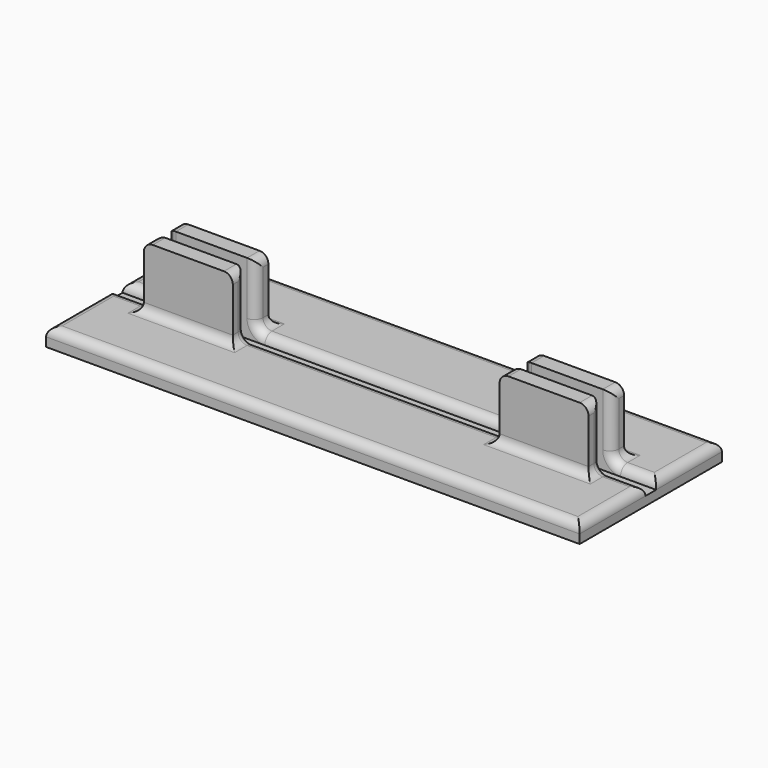
from build123d import *

# Parameters (mm, degrees)
F0_W     = 60
F0_H     = 20
F1_DEPTH = 2
F2_W     = 10
F2_H     = 5
F3_DEPTH = 7
F4_W     = 60
F4_H     = 1.5
F5_DEPTH = 8
F6_F1_R  = 1
F6_F2_R  = 0.9999


# Not quite as in the source:
# - a fillet or chamfer is up to 0.001 mm smaller than in the source, because OpenCascade refuses the exact size


with BuildPart() as f1:
    # F0 (on Top) → F1 (new body)
    with BuildSketch(Plane.XY):
        Rectangle(F0_W, F0_H)
    extrude(amount=F1_DEPTH)

    # F2 (on face) → F3 (join)
    with BuildSketch(Plane.XY.offset(2)):
        with Locations((-20, 0)):
            Rectangle(F2_W, F2_H)
        with Locations((20, 0)):
            Rectangle(F2_W, F2_H)
    extrude(amount=F3_DEPTH)

    # F4 (on face) → F5 (cut)
    with BuildSketch(Plane.XY.offset(9)):
        Rectangle(F4_W, F4_H)
    extrude(amount=-F5_DEPTH, mode=Mode.SUBTRACT)

    # F6: fillet of radius 1 on 32 edges, made by hand

    # F6_f1
    f6_f1_edges = [f1.edges().sort_by_distance(p)[0] for p in [
        (-25, -1.625, 2),
        (-20, -2.5, 2),
        (-15, -1.625, 2),
        (15, -1.625, 2),
        (20, -2.5, 2),
        (25, -1.625, 2),
        (25, 1.625, 2),
        (20, 2.5, 2),
        (15, 1.625, 2),
        (-15, 1.625, 2),
        (-20, 2.5, 2),
        (-25, 1.625, 2),
    ]]
    fillet(f6_f1_edges, radius=F6_F1_R)

    # F6_f2 (radius 1 in the source; OpenCascade refuses exactly that, so slightly less here)
    f6_f2_edges = [f1.edges().sort_by_distance(p)[0] for p in [
        (-15, 1.625, 9),
        (-25, 1.625, 9),
        (-25, -1.625, 9),
        (-15, -1.625, 9),
        (15, 1.625, 9),
        (15, -1.625, 9),
        (25, 1.625, 9),
        (25, -1.625, 9),
        (-28, -0.75, 2),
        (0, -0.75, 2),
        (28, -0.75, 2),
        (30, -5.375, 2),
        (0, -10, 2),
        (-30, -5.375, 2),
        (0, 10, 2),
        (30, 5.375, 2),
        (28, 0.75, 2),
        (0, 0.75, 2),
        (-28, 0.75, 2),
        (-30, 5.375, 2),
        (-25.2928932188, 0.75, 2.2928932188),
        (14.7071067812, 0.75, 2.2928932188),
        (-14.7071067812, 0.75, 2.2928932188),
        (25.2928932188, 0.75, 2.2928932188),
        (25.2928932188, -0.75, 2.2928932188),
        (-14.7071067812, -0.75, 2.2928932188),
        (14.7071067812, -0.75, 2.2928932188),
        (-25.2928932188, -0.75, 2.2928932188),
    ]]
    fillet(f6_f2_edges, radius=F6_F2_R)


solid = f1.part
